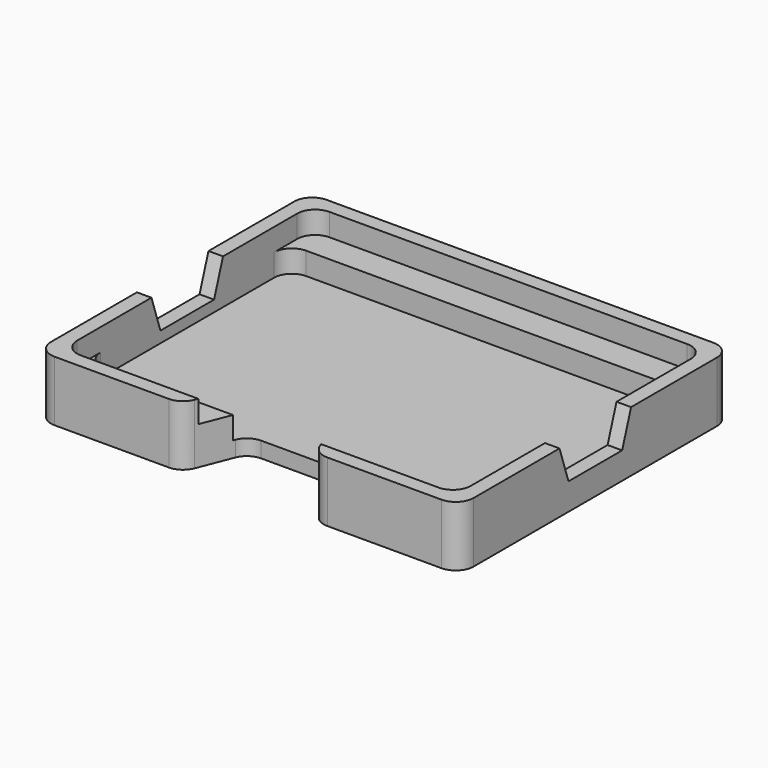
from build123d import *

# Parameters (mm, degrees)
F2_DEPTH      = 3.5
F2_DEPTH_BACK = 10
F3_DEPTH      = 5
F5_START      = 5
F5_DEPTH      = 5
F7_DEPTH      = 10
F7_DEPTH_BACK = 3.5
F8_R          = 4
F10_DEPTH     = 94.501


with BuildPart() as f2:
    # F1 (on Top) → F2 (new body, two sides)
    with BuildSketch(Plane.XY) as f2_sk:
        with BuildLine():
            ThreePointArc((-3.25, -5.75), (-2.0784271247, -8.5784271247), (0.75, -9.75))
            Line((0.75, -9.75), (87.25, -9.75))
            ThreePointArc((87.25, -9.75), (90.0784271247, -8.5784271247), (91.25, -5.75))
            Line((91.25, -5.75), (91.25, 62.25))
            ThreePointArc((91.25, 62.25), (90.0784271247, 65.0784271247), (87.25, 66.25))
            Line((87.25, 66.25), (0.75, 66.25))
            ThreePointArc((0.75, 66.25), (-2.0784271247, 65.0784271247), (-3.25, 62.25))
            Line((-3.25, 62.25), (-3.25, -5.75))
        make_face()
    extrude(amount=-F2_DEPTH)
    extrude(f2_sk.sketch, amount=F2_DEPTH_BACK)

    # F0 (on Top) → F3 (cut)
    with BuildSketch(Plane.XY):
        with BuildLine():
            ThreePointArc((0, 4), (1.1715728753, 1.1715728753), (4, 0))
            Line((4, 0), (84, 0))
            ThreePointArc((84, 0), (86.8284271247, 1.1715728753), (88, 4))
            Line((88, 4), (88, 52.5))
            ThreePointArc((88, 52.5), (86.8284271247, 55.3284271247), (84, 56.5))
            Line((84, 56.5), (4, 56.5))
            ThreePointArc((4, 56.5), (1.1715728753, 55.3284271247), (0, 52.5))
            Line((0, 52.5), (0, 4))
        make_face()
    extrude(amount=F3_DEPTH, mode=Mode.SUBTRACT)

    # F4 (on Top) → F5 (cut)
    with BuildSketch(Plane.XY.offset(F5_START)):
        with BuildLine():
            ThreePointArc((0, -2.5), (1.1715728753, -5.3284271247), (4, -6.5))
            Line((4, -6.5), (84, -6.5))
            ThreePointArc((84, -6.5), (86.8284271247, -5.3284271247), (88, -2.5))
            Line((88, -2.5), (88, 59))
            ThreePointArc((88, 59), (86.8284271247, 61.8284271247), (84, 63))
            Line((84, 63), (4, 63))
            ThreePointArc((4, 63), (1.1715728753, 61.8284271247), (0, 59))
            Line((0, 59), (0, -2.5))
        make_face()
    extrude(amount=F5_DEPTH, mode=Mode.SUBTRACT)

    # F6 (on Top) → F7 (cut, two sides)
    with BuildSketch(Plane.XY) as f7_sk:
        with BuildLine():
            Line((33.0040588687, 0.4603501153), (29, -9.75))
            Line((29, -9.75), (44, -9.75))
            Line((44, -9.75), (59, -9.75))
            Line((59, -9.75), (54.9959411313, 0.4603501153))
            ThreePointArc((54.9959411313, 0.4603501153), (53.5257785273, 2.3046482764), (51.2720483373, 3))
            Line((51.2720483373, 3), (44, 3))
            Line((44, 3), (36.7279516627, 3))
            ThreePointArc((36.7279516627, 3), (34.4742214727, 2.3046482764), (33.0040588687, 0.4603501153))
        make_face()
    extrude(amount=F7_DEPTH, mode=Mode.SUBTRACT)
    extrude(f7_sk.sketch, amount=-F7_DEPTH_BACK, mode=Mode.SUBTRACT)

    # F8
    f8_edges = [f2.edges().sort_by_distance(p)[0] for p in [
        (59, -9.75, 3.25),
        (29, -9.75, 3.25),
    ]]
    fillet(f8_edges, radius=F8_R)

    # F9 (on face) → F10 (cut, through all)
    with BuildSketch(Plane(origin=(-3.25, 0, 0), x_dir=(0, -1, 0), z_dir=(-1, 0, 0))):
        Polygon((-20.75, 2.5), (-18.25, 10), (-28.25, 10), (-38.25, 10), (-35.75, 2.5), (-28.25, 2.5), align=None)
    extrude(amount=-F10_DEPTH, mode=Mode.SUBTRACT)


solid = f2.part
